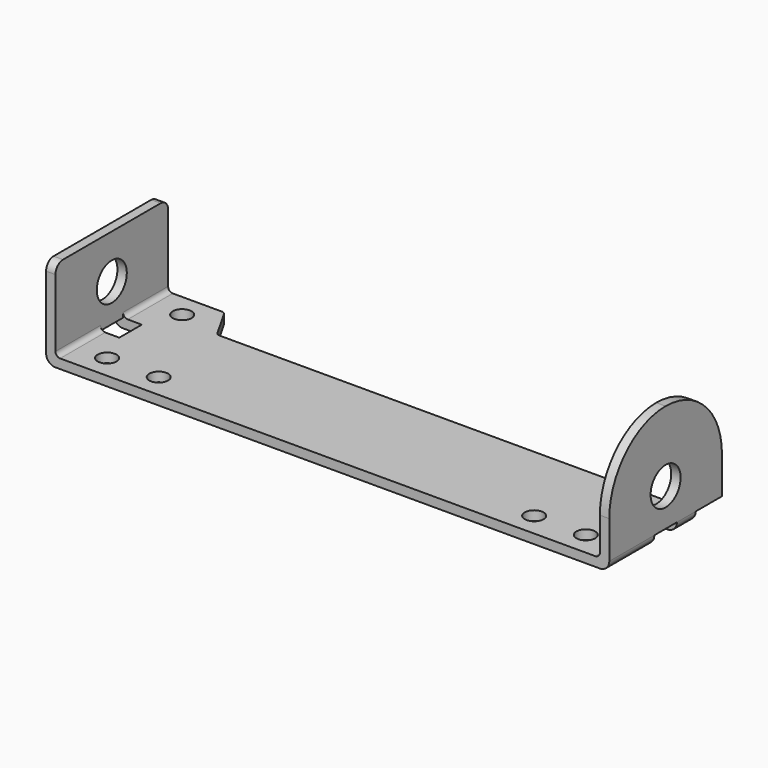
from build123d import *

# Parameters (mm, degrees)
F0_W      = 60
F0_H      = 15
F1_DEPTH  = 1
F2_W      = 1
F2_H      = 15
F3_DEPTH  = 8.7
F4_W      = 1
F4_H      = 15
F5_DEPTH  = 11.5
F6_W      = 3
F6_H      = 3
F6_R      = 1
F7_DEPTH  = 1
F8_R      = 7.49999
F9_R      = 0.5
F10_R     = 1
F11_R     = 2
F12_DEPTH = 60.001


# Not quite as in the source:
# - a fillet or chamfer is up to 0.001 mm smaller than in the source, because OpenCascade refuses the exact size


with BuildPart() as f1:
    # F0 (on Top) → F1 (new body)
    with BuildSketch(Plane.XY):
        with Locations((30, 7.5)):
            Rectangle(F0_W, F0_H)
    extrude(amount=F1_DEPTH)

    # F2 (on face) → F3 (join)
    with BuildSketch(Plane.XY.offset(1)):
        with Locations((0.5, 7.5)):
            Rectangle(F2_W, F2_H)
    extrude(amount=F3_DEPTH)

    # F4 (on face) → F5 (join)
    with BuildSketch(Plane.XY.offset(1)):
        with Locations((59.5, 7.5)):
            Rectangle(F4_W, F4_H)
    extrude(amount=F5_DEPTH)

    # F6 (on face) → F7 (cut, through all)
    with BuildSketch(Plane(origin=(0, 0, 0), x_dir=(1, 0, 0), z_dir=(0, 0, -1))):
        with Locations((1.5, -7.5)):
            Rectangle(F6_W, F6_H)
        with Locations((4.5, -2.5)):
            Circle(F6_R)
        with Locations((10, -2.5)):
            Circle(F6_R)
        with Locations((50, -2.5)):
            Circle(F6_R)
        with Locations((55.5, -2.5)):
            Circle(F6_R)
        with Locations((58.5, -7.5)):
            Rectangle(F6_W, F6_H)
        with Locations((4.5, -12.5)):
            Circle(F6_R)
        Polygon((9, -11.5), (7, -15), (60, -15), (60, -11.5), align=None)
    extrude(amount=-F7_DEPTH, mode=Mode.SUBTRACT)

    # F8 (radius 7.5 in the source; OpenCascade refuses exactly that, so slightly less here)
    f8_edges = [f1.edges().sort_by_distance(p)[0] for p in [
        (59.5, 0, 12.5),
        (59.5, 15, 12.5),
    ]]
    fillet(f8_edges, radius=F8_R)

    # F9
    f9_edges = [f1.edges().sort_by_distance(p)[0] for p in [
        (59, 3, 1),
        (59, 10.25, 1),
        (1, 3, 1),
        (1, 12, 1),
        (7, 15, 0.5),
        (9, 11.5, 0.5),
    ]]
    fillet(f9_edges, radius=F9_R)

    # F10
    f10_edges = [f1.edges().sort_by_distance(p)[0] for p in [
        (60, 10.25, 0),
        (60, 3, 0),
        (0, 12, 0),
        (0, 3, 0),
        (0.5, 0, 9.7),
        (0.5, 15, 9.7),
    ]]
    fillet(f10_edges, radius=F10_R)

    # F11 (on face) → F12 (cut, through all)
    with BuildSketch(Plane.YZ.offset(60)):
        with Locations((7.5, 5)):
            Circle(F11_R)
    extrude(amount=-F12_DEPTH, mode=Mode.SUBTRACT)


solid = f1.part
